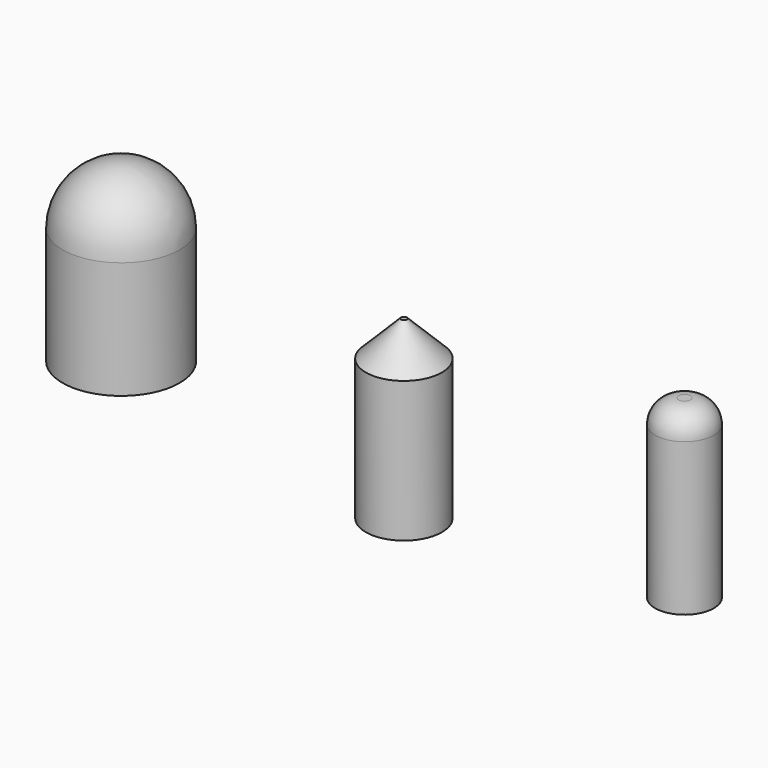
from build123d import *

# Parameters (mm, degrees)
F0_R        = 3.25
F1_DEPTH    = 15
F0_R_2      = 2.5
F0_R_3      = 5
F3_DEPTH    = 10
F4_R        = 0.75
F5_DEPTH    = 10
F6_R        = 5
F7_T2_ANGLE = 359.64
F7_T4_ANGLE = 222.7260056462
F8_R        = 2


# Not quite as in the source:
# - a fillet or chamfer that OpenCascade refuses, or shapes differently, is made with other operations: its cross-section is extruded or revolved along the edge and cut away or added


with BuildPart() as f1:
    # F0 (on Top) → F1 (new body)
    with BuildSketch(Plane.XY):
        Circle(F0_R)
    extrude(amount=F1_DEPTH)

    # F2 (on face) → F3 (cut)
    with BuildSketch(Plane.XY.offset(15)):
        with BuildLine():
            Line((0.1891717111, 0.5198842073), (0.1891717111, 3.2444898002))
            ThreePointArc((0.1891717111, 3.2444898002), (0, 3.25), (-0.1891717111, 3.2444898002))
            Line((-0.1891717111, 3.2444898002), (-0.1891717111, 0.5198842073))
            Line((-0.1891717111, 0.5198842073), (0.1891717111, 0.5198842073))
        make_face()
    extrude(amount=-F3_DEPTH, mode=Mode.SUBTRACT)

    # F7: chamfer of 3 on 2 edges, made by hand

    # F7_s1 → F7_t2 (revolve, cut)
    with BuildSketch(Plane(origin=(0, 0, 0), x_dir=(0, 0, 1), z_dir=(0.006283144, -0.9999802609, 0))):
        Polygon((12, -3.25), (15, -0.25), (15, -3.25), align=None)
    revolve(axis=Axis((0, 0, 15), (0, 0, 1)), revolution_arc=F7_T2_ANGLE, mode=Mode.SUBTRACT)

    # F7_s3 → F7_t4 (revolve, cut)
    with BuildSketch(Plane.XZ):
        Polygon((3.25, 12), (0.25, 15), (3.25, 15), align=None)
    revolve(axis=Axis((0, 0, 15), (0, 0, 1)), revolution_arc=F7_T4_ANGLE, mode=Mode.SUBTRACT)


with BuildPart() as f1b:
    # F0 (on Top) → F1, piece 2 (new body)
    with BuildSketch(Plane.XY):
        with Locations((21.7513348907, 2.7434001677)):
            Circle(F0_R_2)
    extrude(amount=F1_DEPTH)

    # F8
    f8_edges = [f1b.edges().sort_by_distance(p)[0] for p in [
        (19.251335, 2.7434, 15),
    ]]
    fillet(f8_edges, radius=F8_R)


with BuildPart() as f1c:
    # F0 (on Top) → F1, piece 3 (new body)
    with BuildSketch(Plane.XY):
        with Locations((-28.8588888943, 5.9040305205)):
            Circle(F0_R_3)
    extrude(amount=F1_DEPTH)

    # F4 (on Top) → F5 (cut)
    with BuildSketch(Plane.XY):
        with Locations((-28.8588888943, 5.9040305205)):
            Circle(F4_R)
        Circle(F4_R)
        with Locations((21.7513348907, 2.7434001677)):
            Circle(F4_R)
    extrude(amount=F5_DEPTH, mode=Mode.SUBTRACT)

    # F6
    f6_edges = [f1c.edges().sort_by_distance(p)[0] for p in [
        (-33.858889, 5.904031, 15),
    ]]
    fillet(f6_edges, radius=F6_R)


solid = Compound([f1.part, f1b.part, f1c.part])
